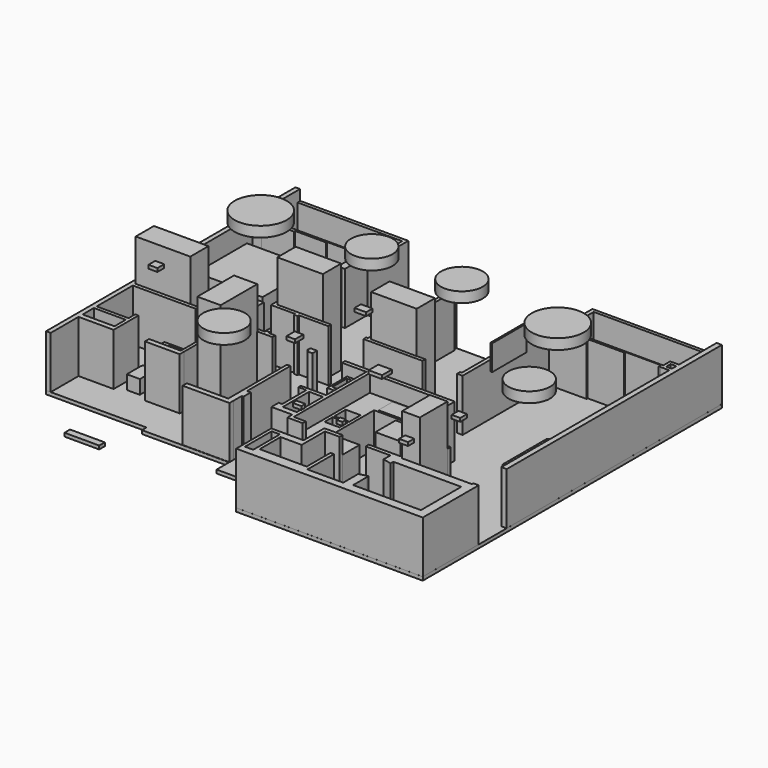
from build123d import *

# Parameters (mm, degrees)
F0_W      = 10
F0_H      = 2
F1_DEPTH  = 1
F3_DEPTH  = 1
F4_W      = 1.7179399729
F4_H      = 0.9254515171
F4_W_2    = 8.9865811169
F4_H_2    = 1.475661993
F4_W_3    = 9.1749764979
F4_H_3    = 0.992551446
F4_W_4    = 18.0843584239
F4_H_4    = 1.0441546328
F4_W_5    = 0.8741877973
F4_H_5    = 18.0519050919
F4_W_6    = 0.5928017199
F4_H_6    = 1.0099140927
F4_W_7    = 1.0744202882
F4_H_7    = 0.4943464883
F4_W_8    = 3.9996404666
F4_H_8    = 1.604065299
F4_W_9    = 2.3124715153
F4_H_9    = 0.8548051119
F4_H_10   = 1.1067464948
F4_W_10   = 5.2964361385
F4_H_11   = 1.1198185384
F4_W_11   = 0.9630378336
F4_H_12   = 0.0292840414
F4_H_13   = 6.840385031
F4_W_12   = 1.072043553
F4_H_14   = 6.3775070012
F4_W_13   = 2.3909630254
F4_H_15   = 9.5941163599
F4_W_14   = 1.5586204827
F4_H_16   = 0.5217976868
F4_W_15   = 1.0914411396
F4_H_17   = 0.4875999875
F4_W_16   = 0.4432513379
F4_H_18   = 1.052968204
F4_W_17   = 0.9357857052
F4_H_19   = 1.0247346945
F4_W_18   = 0.5038850941
F4_W_19   = 15.5666992068
F4_W_20   = 0.5038846284
F4_H_20   = 1.0437616147
F4_W_21   = 1.6494318843
F4_H_21   = 0.9382255375
F5_DEPTH  = 15
F6_W      = 0.9764041752
F6_H      = 15.064522624
F6_W_2    = 34.5774684101
F6_H_2    = 0.9403638542
F7_DEPTH  = 12
F9_DEPTH  = 10
F10_W     = 7.1716625243
F10_H     = 7.3057133704
F11_DEPTH = 18
F12_W     = 5.0494447351
F12_H     = 9.9939070642
F13_DEPTH = 27
F14_W     = 15.6972967088
F14_H     = 6.5492992289
F14_W_2   = 6.7069586366
F14_H_2   = 13.1884724833
F14_W_3   = 13.0917895585
F14_H_3   = 6.5957107581
F14_W_4   = 13.0917887436
F14_H_4   = 6.6261407919
F15_DEPTH = 27
F16_W     = 19.1
F16_H     = 18.3
F17_DEPTH = 9
F18_W     = 4.3041501194
F18_H     = 2.9092859477
F18_H_2   = 4.1005741805
F19_DEPTH = 4
F20_W     = 6.8197827786
F20_H     = 5.0101107918
F21_DEPTH = 0.2
F22_W     = 0.5733296275
F22_H     = 1.0049194098
F22_W_2   = 8.8684801012
F22_H_2   = 0.3130510449
F22_W_3   = 10.3186219931
F22_H_3   = 0.2522543073
F23_DEPTH = 15
F24_W     = 1
F24_H     = 1
F25_DEPTH = 7.2
F27_DEPTH = 0.4
F29_DEPTH = 8
F30_W     = 9.0107955039
F30_H     = 1.475661993
F30_W_2   = 10.0773833692
F30_H_2   = 1.5270002186
F30_W_3   = 8.048088057
F30_H_3   = 2.6454497129
F30_W_4   = 5.3399289027
F30_H_4   = 1.1198185384
F31_DEPTH = 15
F32_W     = 12.32
F32_H     = 7.3
F33_DEPTH = 0.5
F35_DEPTH = 4
F36_W     = 9.1707929969
F36_H     = 5.5558662862
F36_W_2   = 5.594753311
F36_H_2   = 7.2097331285
F37_DEPTH = 12
F38_W     = 5.3351223469
F38_H     = 3.7588365376
F38_W_2   = 3.8315872662
F38_H_2   = 5.2381199785
F39_DEPTH = 2.5
F40_W     = 6.1975358811
F40_H     = 16.8274068087
F41_DEPTH = 4
F42_F1_R  = 1
F42_F2_R  = 1
F44_R     = 7.5
F45_DEPTH = 3
F44_R_2   = 6
F46_W     = 12.7
F46_H     = 7.62
F47_DEPTH = 10
F48_W     = 2.581089735
F48_H     = 2.4520345032
F49_DEPTH = 1
F48_W_2   = 2.4520343868
F48_H_2   = 2.9682535678
F48_W_3   = 3.8716346025
F48_H_3   = 3.4844689071
F48_W_4   = 3.3554165275
F48_H_4   = 2.3229801445
F48_W_5   = 2.4520326406
F48_H_5   = 1.4196000993
F48_W_6   = 1.6777087003
F48_W_7   = 2.5810971856
F48_H_6   = 2.1939240396
F48_W_8   = 2.4520345032
F48_H_7   = 2.4520326406


with BuildPart() as f1:
    # F0 (on Top) → F1 (new body)
    with BuildSketch(Plane.XY):
        with Locations((-39.0686057508, -49.9685147653)):
            Rectangle(F0_W, F0_H)
    extrude(amount=F1_DEPTH)


with BuildPart() as f3:
    # F2 (on Top) → F3 (new body)
    with BuildSketch(Plane.XY):
        Polygon((-28.8841184229, 53.7188947201), (-61.3672323525, 53.7188947201), (-61.3672323525, -35.9670072794), (-32.4498265982, -35.9670072794), (-32.4498265982, -37.6164503396), (-7.3635582812, -37.6164503396), (-7.3635582812, -42.1154238284), (7.7169961296, -42.1154238284), (7.7169961296, -53.9189465344), (61.4204779267, -53.9189465344), (61.4204779267, 53.7188947201), (24.1786744446, 53.7188947201), (24.1786744446, 37.7183668315), (-28.8841184229, 37.7183668315), align=None)
    extrude(amount=-F3_DEPTH)

    # F4 (on Top) → F5 (join)
    with BuildSketch(Plane.XY):
        Polygon((-60.0302144885, 53.7365972996), (-61.3627694547, 53.7365972996), (-61.3627694547, -35.9646901488), (-60.0302144885, -35.9646901488), (-60.0302144885, -25.9622130543), (-60.0302144885, -24.4865510613), (-60.0302144885, -20.4392336309), (-60.0302144885, -19.4466821849), (-60.0302144885, -6.4334324561), (-60.0302144885, -5.3892778233), (-60.0302144885, 36.7141552269), (-60.0302144885, 37.6396067441), (-60.0302144885, 39.2337068915), (-60.0302144885, 40.1499085128), align=None)
        Polygon((-57.4978739023, 40.1499085128), (-60.0302144885, 40.1499085128), (-60.0302144885, 39.2337068915), (-58.3122745156, 39.2337068915), (-57.4978739023, 39.2337068915), align=None)
        Polygon((-60.0302144885, -24.4865510613), (-60.0302144885, -25.9622130543), (-49.923337996, -25.9622130543), (-49.923337996, -24.4865510613), (-50.8552379906, -24.4865510613), align=None)
        with Locations((-59.1712445021, 37.1768809855)):
            Rectangle(F4_W, F4_H)
        Polygon((-57.4978739023, 39.2337068915), (-58.3122745156, 39.2337068915), (-58.3122745156, 37.6396067441), (-58.3122745156, 36.7141552269), (-57.4978739023, 36.7141552269), align=None)
        with Locations((-45.4300474375, -25.2243820578)):
            Rectangle(F4_W_2, F4_H_2)
        with Locations((-55.4427262396, -19.9429579079)):
            Rectangle(F4_W_3, F4_H_3)
        Polygon((-50.8552379906, -20.4392336309), (-50.8552379906, -24.4865510613), (-49.923337996, -24.4865510613), (-49.923337996, -17.0543789864), (-50.8552379906, -17.0543789864), (-50.8552379906, -19.4466821849), align=None)
        Polygon((-40.9367568791, -24.4865510613), (-40.9367568791, -25.9622130543), (-32.371416688, -25.9622130543), (-30.9110619128, -25.9622130543), (-30.9110619128, -24.4747549295), (-31.7852497101, -24.4747549295), (-40.9367568791, -24.4747549295), align=None)
        with Locations((-50.9880352765, -5.9113551397)):
            Rectangle(F4_W_4, F4_H_4)
        Polygon((-30.9110619128, -25.9622130543), (-32.371416688, -25.9622130543), (-32.371416688, -35.9872579575), (-32.371416688, -37.5142581761), (-20.8478253335, -37.5142581761), (-20.8478253335, -35.9872579575), (-30.9110619128, -35.9872579575), align=None)
        with Locations((-31.3481558114, -15.4488023836)):
            Rectangle(F4_W_5, F4_H_5)
        with Locations((-32.08165057, -5.9178927913)):
            Rectangle(F4_W_6, F4_H_6)
        with Locations((-31.3481558114, -5.9178927913)):
            Rectangle(F4_W_5, F4_H_6)
        Polygon((-30.9110619128, -5.412935745), (-30.9110619128, -6.4228498377), (-19.8330618441, -6.4228498377), (-19.8330618441, -5.412935745), (-21.8003112823, -5.412935745), (-22.8747315705, -5.412935745), align=None)
        Polygon((-8.912473917, -35.9872579575), (-20.8478253335, -35.9872579575), (-20.8478253335, -37.5142581761), (-7.3338598013, -37.5142581761), (-7.3338598013, -35.9872579575), (-7.9137170687, -35.9872579575), align=None)
        Polygon((-8.912473917, -14.8792490363), (-8.912473917, -35.9872579575), (-7.9137170687, -35.9872579575), (-7.9137170687, -30.4961726069), (-7.9137170687, -14.8792490363), align=None)
        with Locations((-22.3375214264, -5.1657625008)):
            Rectangle(F4_W_7, F4_H_7)
        Polygon((-7.9137170687, -30.4961726069), (-7.9137170687, -35.9872579575), (-7.3338598013, -35.9872579575), (-7.3084095493, -33.1292562187), (-6.8241641857, -33.1292562187), (1.2239238713, -33.1168919802), (3.2214371022, -33.1168919802), (3.2214371022, -31.5128266811), (3.2214371022, -30.4838065058), (2.2226804867, -30.4838065058), (1.2239238713, -30.4838065058), (-6.8241641857, -30.4961726069), align=None)
        Polygon((2.2226804867, -21.8050256371), (2.2226804867, -30.4838065058), (3.2214371022, -30.4838065058), (3.2214371022, -22.05696702), (3.2214371022, -20.9502205253), (2.2226804867, -20.9502205253), align=None)
        with Locations((5.2212573355, -32.3148593307)):
            Rectangle(F4_W_8, F4_H_8)
        with Locations((1.0664447291, -21.3776230812)):
            Rectangle(F4_W_9, F4_H_9)
        Polygon((7.2210775688, -31.5128266811), (7.2210775688, -33.1168919802), (7.2210775688, -33.7888039649), (8.1849554554, -33.7888039649), (8.1849554554, -6.4228498377), (7.2210775688, -6.4228498377), (7.2210775688, -20.9502205253), (7.2210775688, -22.05696702), align=None)
        with Locations((5.2212573355, -21.5035937726)):
            Rectangle(F4_W_8, F4_H_10)
        Polygon((8.1849554554, -33.7888039649), (7.2210775688, -33.7888039649), (7.2210775688, -34.9086225033), (11.7003498599, -34.9086225033), (11.7003498599, -33.7888039649), align=None)
        with Locations((14.3485679291, -34.3487132341)):
            Rectangle(F4_W_10, F4_H_11)
        Polygon((7.2210775688, -6.4228498377), (8.1849554554, -6.4228498377), (30.785838142, -6.4228498377), (30.785838142, -6.3935657963), (31.7488759756, -6.3935657963), (31.7488759756, -5.3222225979), (0.1850503613, -5.3222225979), (0.1850503613, -6.4228498377), align=None)
        Polygon((22.2629588097, -33.7888039649), (16.9967859983, -33.7888039649), (16.9967859983, -34.9086225033), (18.0688295513, -34.9086225033), (22.2629588097, -34.9086225033), align=None)
        with Locations((31.2673570588, -6.408207817)):
            Rectangle(F4_W_11, F4_H_12)
        with Locations((31.2673570588, -9.8430423532)):
            Rectangle(F4_W_11, F4_H_13)
        with Locations((17.5328077748, -38.0973760039)):
            Rectangle(F4_W_12, F4_H_14)
        Polygon((18.0688295513, -41.2861295044), (16.9967859983, -41.2861295044), (7.7180769295, -41.2861295044), (7.7180769295, -53.9065264165), (36.8395522237, -53.9065264165), (36.8395522237, -51.8184714019), (26.5431273729, -51.8184714019), (26.5431273729, -42.284887284), (25.5443714559, -42.284887284), (25.5443714559, -50.8197173476), (11.9854928926, -50.8197173476), (11.9854928926, -43.2836413383), (18.0688295513, -43.2836413383), align=None)
        with Locations((9.8517858423, -47.1424739808)):
            Rectangle(F4_W_13, F4_H_15, mode=Mode.SUBTRACT)
        Polygon((36.8395522237, -51.8184714019), (36.8395522237, -53.9065264165), (61.4177882671, -53.9065264165), (61.4177882671, -51.3384267688), (58.8329024613, -51.3384267688), (39.322052151, -51.3384267688), (36.8395522237, -51.3384267688), align=None)
        Polygon((58.8329024613, -51.3384267688), (61.4177882671, -51.3384267688), (61.4177882671, -34.3076325953), (59.8591677845, -34.3076325953), (58.8329024613, -34.3076325953), (58.8329024613, -36.8312001228), align=None)
        Polygon((36.8395522237, -46.4401766658), (36.8395522237, -51.3384267688), (39.322052151, -51.3384267688), (39.322052151, -46.4401766658), (39.3211826014, -45.7283685133), align=None)
        with Locations((60.6384780258, -34.0467337519)):
            Rectangle(F4_W_14, F4_H_16)
        Polygon((39.3103137612, -36.8312001228), (58.8329024613, -36.8312001228), (58.8329024613, -34.3076325953), (39.8210547864, -34.3076325953), (36.8395522237, -34.3076325953), (36.8395522237, -34.8561704159), (36.8395522237, -36.8312001228), (36.8395522237, -37.2750237584), (39.3103137612, -37.8314480186), align=None)
        Polygon((36.8395522237, -34.3076325953), (39.8210547864, -34.3076325953), (39.8210547864, -24.3198573589), (44.8601581156, -24.3198573589), (44.8601581156, -23.1746062636), (31.7788459361, -23.1746062636), (31.7788459361, -22.207506001), (30.7353939861, -22.2329553217), (30.7353939861, -24.3198573589), (38.8285033405, -24.3198573589), (38.8285033405, -33.7618179619), (29.7682937235, -33.7618179619), (29.7682937235, -34.8561704159), (36.8395522237, -34.8561704159), align=None)
        Polygon((-27.8612263501, 37.7254001796), (-29.8767667264, 37.7254001796), (-29.8767667264, 29.6632423997), (-28.8689965382, 29.6632423997), (-27.8612263501, 29.6632423997), align=None)
        Polygon((-28.8689965382, 29.6632423997), (-29.8767667264, 29.6632423997), (-29.8767667264, 5.5812005885), (-28.8689965382, 5.5812005885), (-28.8689965382, 6.5992018208), align=None)
        Polygon((-13.3584560826, 6.5992018208), (-28.8689965382, 6.5992018208), (-28.8689965382, 5.5812005885), (-22.9007676244, 5.5812005885), (-21.8093264848, 5.5812005885), (-13.3584560826, 5.5812005885), align=None)
        with Locations((-22.3550470546, 5.3374005947)):
            Rectangle(F4_W_15, F4_H_17)
        Polygon((-2.5854285341, 36.6724319756), (-2.7778598014, 36.6724319756), (-2.7778598014, 6.6362651996), (-1.8420740962, 6.6362651996), (-1.8420740962, 36.6724319756), (-2.1421771962, 36.6724319756), align=None)
        with Locations((-2.3638028651, 37.1989160776)):
            Rectangle(F4_W_16, F4_H_18)
        with Locations((-2.3099669488, 6.1238978524)):
            Rectangle(F4_W_17, F4_H_19)
        with Locations((-3.0298023485, 6.1238978524)):
            Rectangle(F4_W_18, F4_H_19)
        with Locations((5.9412755072, 6.1238978524)):
            Rectangle(F4_W_19, F4_H_19)
        Polygon((25.2904798836, 29.6683628112), (25.2904798836, 37.7360209823), (23.2544783503, 37.7360209823), (23.2544783503, 29.6683628112), (24.2215543985, 29.6683628112), align=None)
        Polygon((25.2904798836, 5.5698822252), (25.2904798836, 29.6683628112), (24.2215543985, 29.6683628112), (24.2215543985, 6.61364384), (24.2215543985, 5.5698822252), align=None)
        with Locations((23.9696120843, 6.0917630326)):
            Rectangle(F4_W_20, F4_H_20)
        Polygon((61.4177882671, -23.7201843411), (61.4177882671, 53.7296496332), (59.8877593875, 53.7296496332), (59.8877593875, 40.1953980327), (59.8877593875, 39.2269082367), (59.8877593875, 37.6228429377), (59.8877593875, 36.6846174002), (59.8877593875, -23.7201843411), align=None)
        Polygon((59.8877593875, 39.2269082367), (59.8877593875, 40.1953980327), (57.3606342077, 40.1953980327), (57.3606342077, 39.2269082367), (58.2383275032, 39.2269082367), align=None)
        with Locations((59.0630434453, 37.1537301689)):
            Rectangle(F4_W_21, F4_H_21)
        Polygon((58.2383275032, 37.6228429377), (58.2383275032, 39.2269082367), (57.3606342077, 39.2269082367), (57.3606342077, 36.6846174002), (58.2383275032, 36.6846174002), align=None)
        Polygon((-7.8859189525, -6.9533986971), (-7.8859189525, -5.3222225979), (-9.7988750786, -5.3222225979), (-9.7988750786, -6.4353067428), (-9.3405628577, -6.4353067428), (-9.3405628577, -6.9533986971), align=None)
    extrude(amount=F5_DEPTH)

    # F6 (on Top) → F7 (join)
    with BuildSketch(Plane.XY):
        Polygon((-28.8755502552, 53.7493489683), (-59.9627941847, 53.7493489683), (-59.9627941847, 52.7634248137), (-29.8519544303, 52.7634248137), (-28.8755502552, 52.7634248137), align=None)
        with Locations((-29.3637523428, 45.2311635017)):
            Rectangle(F6_W, F6_H)
        Polygon((24.1630878299, 53.7037886679), (24.1630878299, 37.6989021897), (25.2903085202, 37.6989021897), (25.2903085202, 52.7634248137), (25.2903085202, 53.7037886679), align=None)
        with Locations((42.5790427253, 53.2336067408)):
            Rectangle(F6_W_2, F6_H_2)
    extrude(amount=F7_DEPTH)

    # F8 (on Top) → F9 (join)
    with BuildSketch(Plane.XY):
        Polygon((8.1922709942, -33.7576754391), (22.2436320037, -33.7576754391), (22.2436320037, -27.6425071061), (14.2403719947, -27.6425071061), (14.2403719947, -12.453218922), (30.8089852333, -12.453218922), (30.8089852333, -6.4128474332), (8.1922709942, -6.4128474332), align=None)
    extrude(amount=F9_DEPTH)

    # F10 (on Top) → F11 (join)
    with BuildSketch(Plane.XY):
        with Locations((34.3118710443, -28.9391381666)):
            Rectangle(F10_W, F10_H)
    extrude(amount=F11_DEPTH)

    # F12 (on Top) → F13 (join)
    with BuildSketch(Plane.XY):
        with Locations((42.3537157476, -29.3100457639)):
            Rectangle(F12_W, F12_H)
    extrude(amount=F13_DEPTH)

    # F14 (on Top) → F15 (join)
    with BuildSketch(Plane.XY):
        with Locations((-52.1805789322, -2.1062588785)):
            Rectangle(F14_W, F14_H)
        with Locations((-27.5712059811, -12.9952195566)):
            Rectangle(F14_W_2, F14_H_2)
        with Locations((-22.2929241136, 9.8818715196)):
            Rectangle(F14_W_3, F14_H_3)
        with Locations((4.7222128487, 9.8970865365)):
            Rectangle(F14_W_4, F14_H_4)
    extrude(amount=F15_DEPTH)

    # F16 (on Top) → F17 (join)
    with BuildSketch(Plane.XY):
        with Locations((-50.4802144885, 25.4931322396)):
            Rectangle(F16_W, F16_H)
    extrude(amount=F17_DEPTH)

    # F18 (on face) → F19 (cut)
    with BuildSketch(Plane.XY.offset(10)):
        with Locations((11.2386140972, -22.3775943741)):
            Rectangle(F18_W, F18_H)
        with Locations((11.2386140972, -18.270556815)):
            Rectangle(F18_W, F18_H_2)
    extrude(amount=-F19_DEPTH, mode=Mode.SUBTRACT)

    # F20 (on face) → F21 (join)
    with BuildSketch(Plane.XY.offset(10)):
        with Locations((18.6193669215, -9.6318901051)):
            Rectangle(F20_W, F20_H)
    extrude(amount=F21_DEPTH)

    # F22 (on Top) → F23 (join)
    with BuildSketch(Plane.XY):
        Polygon((-48.11488837, 37.7053394914), (-56.9423809648, 37.7053394914), (-56.9423809648, 36.7004200816), (-48.11488837, 36.7004200816), (-48.11488837, 37.08358109), align=None)
        with Locations((-57.2290457785, 37.2028797865)):
            Rectangle(F22_W, F22_H)
        Polygon((-39.2455086112, 37.7053394914), (-48.11488837, 37.7053394914), (-48.11488837, 37.08358109), (-39.2455086112, 37.08358109), (-39.2455086112, 37.3922884464), align=None)
        with Locations((-34.8112685606, 37.5488139689)):
            Rectangle(F22_W_2, F22_H_2)
        Polygon((-29.8687852919, 37.7053394914), (-30.37702851, 37.7053394914), (-30.37702851, 37.3922884464), (-30.37702851, 36.7004200816), (-29.8687852919, 36.7004200816), align=None)
        Polygon((25.7350783795, 37.745591253), (25.2841897309, 37.745591253), (25.2841897309, 36.6606414318), (25.7350783795, 36.6606414318), (25.7350783795, 37.6997888088), align=None)
        Polygon((36.1002385616, 37.6997888088), (25.7350783795, 37.6997888088), (25.7350783795, 36.6606414318), (36.1002385616, 36.6606414318), (36.1002385616, 37.0687991381), align=None)
        Polygon((46.5151965618, 37.6997888088), (36.1002385616, 37.6997888088), (36.1002385616, 37.0687991381), (46.5151965618, 37.0687991381), (46.5151965618, 37.4475345016), align=None)
        with Locations((51.6745075583, 37.5736616552)):
            Rectangle(F22_W_3, F22_H_3)
        Polygon((57.3620870709, 37.6997888088), (56.8338185549, 37.6997888088), (56.8338185549, 37.4475345016), (56.8338185549, 36.6879627109), (57.3620870709, 36.6879627109), align=None)
    extrude(amount=F23_DEPTH)

    # F24 (on Top) → F25 (join)
    with BuildSketch(Plane.XY):
        with Locations((50.8877593875, 4.2798156589)):
            Rectangle(F24_W, F24_H)
        with Locations((59.3877593875, 4.2798156589)):
            Rectangle(F24_W, F24_H)
        with Locations((59.3877593875, -11.2201843411)):
            Rectangle(F24_W, F24_H)
        with Locations((50.8877593875, -11.2201843411)):
            Rectangle(F24_W, F24_H)
    extrude(amount=F25_DEPTH)

    # F26 (on face) → F27 (join)
    with BuildSketch(Plane.XY.offset(7.2)):
        with BuildLine():
            ThreePointArc((50.3877593875, -11.2201843411), (50.5342059969, -11.5737377317), (50.8877593875, -11.7201843411))
            Line((50.8877593875, -11.7201843411), (59.3877593875, -11.7201843411))
            ThreePointArc((59.3877593875, -11.7201843411), (59.7413127781, -11.5737377317), (59.8877593875, -11.2201843411))
            Line((59.8877593875, -11.2201843411), (59.8877593875, 4.2798156589))
            ThreePointArc((59.8877593875, 4.2798156589), (59.7413127781, 4.6333690495), (59.3877593875, 4.7798156589))
            Line((59.3877593875, 4.7798156589), (50.8877593875, 4.7798156589))
            ThreePointArc((50.8877593875, 4.7798156589), (50.5342059969, 4.6333690495), (50.3877593875, 4.2798156589))
            Line((50.3877593875, 4.2798156589), (50.3877593875, -11.2201843411))
        make_face()
    extrude(amount=F27_DEPTH)

    # F28 (on Top) → F29 (join)
    with BuildSketch(Plane.XY):
        with BuildLine():
            Line((59.8877593875, 10.6846174002), (59.8877593875, 33.6846174002))
            Line((59.8877593875, 33.6846174002), (51.8877593875, 33.6846174002))
            ThreePointArc((51.8877593875, 33.6846174002), (51.1806526063, 33.3917241814), (50.8877593875, 32.6846174002))
            Line((50.8877593875, 32.6846174002), (50.8877593875, 11.6846174002))
            ThreePointArc((50.8877593875, 11.6846174002), (51.1806526063, 10.977510619), (51.8877593875, 10.6846174002))
            Line((51.8877593875, 10.6846174002), (59.8877593875, 10.6846174002))
        make_face()
    extrude(amount=F29_DEPTH)

    # F30 (on face) → F31 (cut)
    with BuildSketch(Plane.XY.offset(15)):
        with Locations((-45.4179402441, -25.2243820578)):
            Rectangle(F30_W, F30_H)
        Polygon((-30.9110619128, -25.9622130543), (-32.371416688, -25.9622130543), (-32.371416688, -37.5142581761), (-30.9110619128, -37.5142581761), (-30.9110619128, -35.9872579575), align=None)
        with Locations((-25.8723702282, -36.7507580668)):
            Rectangle(F30_W_2, F30_H_2)
        with Locations((-2.8001201572, -31.8065313622)):
            Rectangle(F30_W_3, F30_H_3)
        with Locations((14.326821547, -34.3487132341)):
            Rectangle(F30_W_4, F30_H_4)
    extrude(amount=-F31_DEPTH, mode=Mode.SUBTRACT)

    # F32 (on face) → F33 (join)
    with BuildSketch(Plane.YZ.offset(25.2904798836)):
        with Locations((21.7298822252, 15.65)):
            Rectangle(F32_W, F32_H)
    extrude(amount=F33_DEPTH)

    # F34 (on Top) → F35 (join)
    with BuildSketch(Plane.XY):
        with BuildLine():
            Line((-47.3037548363, -19.6383856237), (-47.3037548363, -24.4917310774))
            Line((-47.3037548363, -24.4917310774), (-43.5515902936, -24.4917310774))
            Line((-43.5515902936, -24.4917310774), (-43.5515902936, -19.6383856237))
            ThreePointArc((-43.5515902936, -19.6383856237), (-45.427672565, -17.7623033524), (-47.3037548363, -19.6383856237))
        make_face()
        with BuildLine():
            Line((7.1799810976, -19.0876163542), (7.1799810976, -15.3151145205))
            Line((7.1799810976, -15.3151145205), (2.3786171805, -15.3151145205))
            ThreePointArc((2.3786171805, -15.3151145205), (0.4923662636, -17.2013654374), (2.3786171805, -19.0876163542))
            Line((2.3786171805, -19.0876163542), (7.1799810976, -19.0876163542))
        make_face()
    extrude(amount=F35_DEPTH)

    # F36 (on Top) → F37 (join)
    with BuildSketch(Plane.XY):
        with Locations((-36.3587737083, -21.7295745388)):
            Rectangle(F36_W, F36_H)
        with Locations((4.4236836839, -9.9426386878)):
            Rectangle(F36_W_2, F36_H_2)
    extrude(amount=F37_DEPTH)

    # F38 (on face) → F39 (cut)
    with BuildSketch(Plane.XY.offset(12)):
        with Locations((-36.4038385451, -21.3321726769)):
            Rectangle(F38_W, F38_H)
        with Locations((4.1528551374, -9.8888499197)):
            Rectangle(F38_W_2, F38_H_2)
    extrude(amount=-F39_DEPTH, mode=Mode.SUBTRACT)

    # F40 (on face) → F41 (cut)
    with BuildSketch(Plane.XY.offset(8)):
        with Locations((53.9865273281, 22.0983208045)):
            Rectangle(F40_W, F40_H)
    extrude(amount=-F41_DEPTH, mode=Mode.SUBTRACT)

    # F42: fillet of radius 1 on 11 edges, made by hand

    # F42_f1
    f42_f1_edges = [f3.edges().sort_by_distance(p)[0] for p in [
        (57.0852952686, 30.5120242089, 6),
        (53.9865273281, 30.5120242089, 4),
        (57.0852952686, 13.6846174002, 6),
        (53.9865273281, 13.6846174002, 4),
        (57.0852952686, 22.0983208045, 4),
    ]]
    fillet(f42_f1_edges, radius=F42_F1_R)

    # F42_f2
    f42_f2_edges = [f3.edges().sort_by_distance(p)[0] for p in [
        (50.8877593875, 30.5120242089, 6.5),
        (53.4865273281, 30.5120242089, 8),
        (50.8877593875, 13.6846174002, 6.5),
        (53.4865273281, 13.6846174002, 8),
        (55.8877593875, 33.6846174002, 8),
        (55.8877593875, 10.6846174002, 8),
        (51.1806526063, 10.977510619, 8),
        (50.8877593875, 12.6846174002, 8),
        (51.1806526063, 33.3917241814, 8),
        (50.8877593875, 31.5983208045, 8),
        (56.7924020498, 13.977510619, 8),
        (50.8877593875, 13.977510619, 4.2928932188),
        (56.7924020498, 30.2191309901, 8),
        (50.8877593875, 30.2191309901, 4.2928932188),
    ]]
    fillet(f42_f2_edges, radius=F42_F2_R)

    # F46 (on face) → F47 (join)
    with BuildSketch(Plane.XY):
        with Locations((-44.2563550711, 9.2748043588)):
            Rectangle(F46_W, F46_H)
    extrude(amount=F47_DEPTH)


with BuildPart() as f45:
    # F44 (on offset) → F45 (new body)
    with BuildSketch(Plane.XY.offset(27)):
        with Locations((-46.0302144885, 22.08358109)):
            Circle(F44_R)
    extrude(amount=-F45_DEPTH)


with BuildPart() as f45b:
    # F44 (on offset) → F45, piece 2 (new body)
    with BuildSketch(Plane.XY.offset(27)):
        with Locations((-15.5778598014, 23.9992018208)):
            Circle(F44_R_2)
    extrude(amount=-F45_DEPTH)


with BuildPart() as f45c:
    # F44 (on offset) → F45, piece 3 (new body)
    with BuildSketch(Plane.XY.offset(27)):
        with Locations((10.1579259038, 24.2362651996)):
            Circle(F44_R_2)
    extrude(amount=-F45_DEPTH)


with BuildPart() as f45d:
    # F44 (on offset) → F45, piece 4 (new body)
    with BuildSketch(Plane.XY.offset(27)):
        with Locations((40.2904798836, 21.0687991381)):
            Circle(F44_R)
    extrude(amount=-F45_DEPTH)


with BuildPart() as f45e:
    # F44 (on offset) → F45, piece 5 (new body)
    with BuildSketch(Plane.XY.offset(27)):
        with Locations((52.3877593875, -4.3076325953)):
            Circle(F44_R_2)
    extrude(amount=-F45_DEPTH)


with BuildPart() as f45f:
    # F44 (on offset) → F45, piece 6 (new body)
    with BuildSketch(Plane.XY.offset(27)):
        with Locations((-18.912473917, -24.9872579575)):
            Circle(F44_R_2)
    extrude(amount=-F45_DEPTH)


with BuildPart() as f49:
    # F48 (on offset) → F49 (new body)
    with BuildSketch(Plane.XY.offset(27)):
        with Locations((-47.9171089828, -13.1192998961)):
            Rectangle(F48_W, F48_H)
    extrude(amount=-F49_DEPTH)


with BuildPart() as f49b:
    # F48 (on offset) → F49, piece 2 (new body)
    with BuildSketch(Plane.XY.offset(27)):
        with Locations((-2.0382488729, -20.6044586375)):
            Rectangle(F48_W_2, F48_H_2)
    extrude(amount=-F49_DEPTH)


with BuildPart() as f49c:
    # F48 (on offset) → F49, piece 3 (new body)
    with BuildSketch(Plane.XY.offset(27)):
        with Locations((23.4500076622, -21.7659492046)):
            Rectangle(F48_W_3, F48_H_3)
    extrude(amount=-F49_DEPTH)


with BuildPart() as f49d:
    # F48 (on offset) → F49, piece 4 (new body)
    with BuildSketch(Plane.XY.offset(27)):
        with Locations((1.7688579101, -0.6655437464)):
            Rectangle(F48_W_4, F48_H_4)
    extrude(amount=-F49_DEPTH)


with BuildPart() as f49e:
    # F48 (on offset) → F49, piece 5 (new body)
    with BuildSketch(Plane.XY.offset(27)):
        with Locations((19.3847911432, -45.8991322666)):
            Rectangle(F48_W_5, F48_H_5)
    extrude(amount=-F49_DEPTH)


with BuildPart() as f49f:
    # F48 (on offset) → F49, piece 6 (new body)
    with BuildSketch(Plane.XY.offset(27)):
        with Locations((31.7740207538, -46.1572427303)):
            Rectangle(F48_W_6, F48_H_5)
    extrude(amount=-F49_DEPTH)


with BuildPart() as f49g:
    # F48 (on offset) → F49, piece 7 (new body)
    with BuildSketch(Plane.XY.offset(27)):
        with Locations((49.0027926862, -44.221425429)):
            Rectangle(F48_W_7, F48_H_6)
    extrude(amount=-F49_DEPTH)


with BuildPart() as f49h:
    # F48 (on offset) → F49, piece 8 (new body)
    with BuildSketch(Plane.XY.offset(27)):
        with Locations((50.8740786463, -27.5734001771)):
            Rectangle(F48_W_8, F48_H_7)
    extrude(amount=-F49_DEPTH)


solid = Compound([f1.part, f3.part, f45.part, f45b.part, f45c.part, f45d.part, f45e.part, f45f.part, f49.part, f49b.part, f49c.part, f49d.part, f49e.part, f49f.part, f49g.part, f49h.part])
